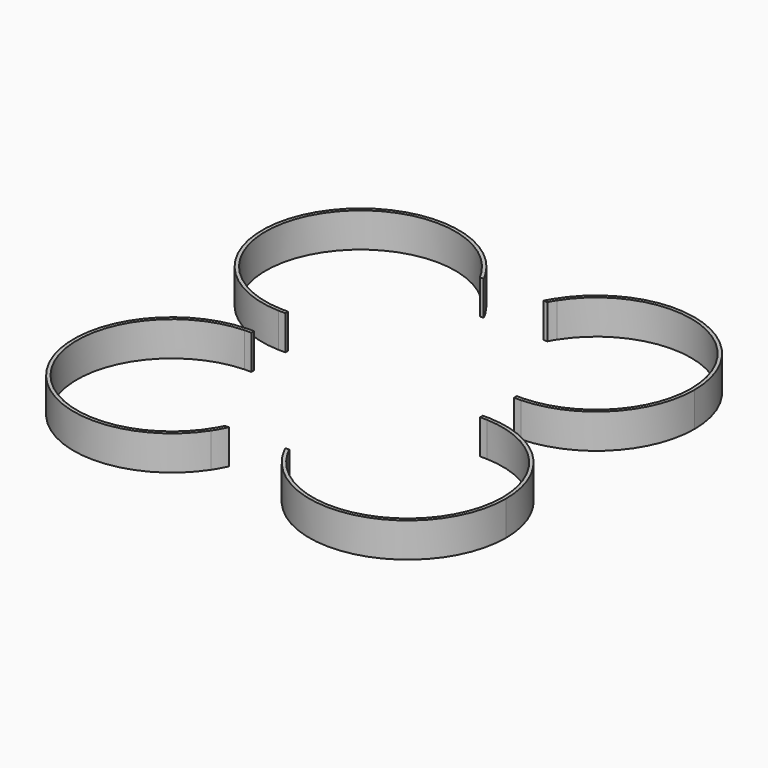
from build123d import *

# Parameters (mm, degrees)
F1_DEPTH = 10


with BuildPart() as f1:
    # F0 (on Top) → F1 (new body)
    with BuildSketch(Plane.XY):
        with BuildLine():
            ThreePointArc((-35.1387531032, -6.6569409359), (-34.1387531032, -6.6387531032), (-33.1387531032, -6.6569409359))
            Line((-33.1387531032, -6.6569409359), (-33.1387531032, -5.6563023659))
            ThreePointArc((-33.1387531032, -5.6563023659), (-34.1387531032, -5.6387531032), (-35.1387531032, -5.6563023659))
            Line((-35.1387531032, -5.6563023659), (-35.1387531032, -6.6569409359))
        make_face()
        with BuildLine():
            Line((-8.2170735426, -45.9842808987), (-9.3207461074, -45.9842808987))
            ThreePointArc((-9.3207461074, -45.9842808987), (-9.8032628947, -46.9463257191), (-10.3230544991, -47.8887531032))
            Line((-10.3230544991, -47.8887531032), (-10.3230544991, -49.7932253077))
            ThreePointArc((-10.3230544991, -49.7932253077), (-9.1972473136, -47.9290137587), (-8.2170735426, -45.9842808987))
        make_face()
        with BuildLine():
            ThreePointArc((-10.3230544991, -47.8887531032), (-57.7004722542, -48.3195637518), (-35.1387531032, -6.6569409359))
            Line((-35.1387531032, -6.6569409359), (-35.1387531032, -5.6563023659))
            ThreePointArc((-35.1387531032, -5.6563023659), (-58.9813781132, -48.1063578589), (-10.3230544991, -49.7932253077))
            Line((-10.3230544991, -49.7932253077), (-10.3230544991, -47.8887531032))
        make_face()
    extrude(amount=F1_DEPTH)


with BuildPart() as f1b:
    # F0 (on Top) → F1, piece 2 (new body)
    with BuildSketch(Plane.XY):
        with BuildLine():
            Line((9.3207461074, -45.9842808987), (8.2170735426, -45.9842808987))
            ThreePointArc((8.2170735426, -45.9842808987), (9.1972473136, -47.9290137587), (10.3230544991, -49.7932253077))
            Line((10.3230544991, -49.7932253077), (10.3230544991, -47.8887531032))
            ThreePointArc((10.3230544991, -47.8887531032), (9.8032628947, -46.9463257191), (9.3207461074, -45.9842808987))
        make_face()
        with BuildLine():
            Line((10.3230544991, -47.8887531032), (10.3230544991, -49.7932253077))
            ThreePointArc((10.3230544991, -49.7932253077), (42.3088996681, -61.4425752735), (62.6387531032, -34.1387531032))
            ThreePointArc((62.6387531032, -34.1387531032), (54.641801657, -14.3429202084), (35.1387531032, -5.6563023659))
            Line((35.1387531032, -5.6563023659), (35.1387531032, -6.6569409359))
            ThreePointArc((35.1387531032, -6.6569409359), (53.934585998, -15.0501439344), (61.6387531032, -34.1387531032))
            ThreePointArc((61.6387531032, -34.1387531032), (41.2562768435, -60.7017133261), (10.3230544991, -47.8887531032))
        make_face()
        with BuildLine():
            Line((35.1387531032, -5.6563023659), (33.1387531032, -5.6563023659))
            Line((33.1387531032, -5.6563023659), (33.1387531032, -6.6569409359))
            ThreePointArc((33.1387531032, -6.6569409359), (34.1387531032, -6.6387531032), (35.1387531032, -6.6569409359))
            Line((35.1387531032, -6.6569409359), (35.1387531032, -5.6563023659))
        make_face()
    extrude(amount=F1_DEPTH)


with BuildPart() as f1c:
    # F0 (on Top) → F1, piece 3 (new body)
    with BuildSketch(Plane.XY):
        with BuildLine():
            Line((-35.1387531032, 5.6563023659), (-33.1387531032, 5.6563023659))
            Line((-33.1387531032, 5.6563023659), (-33.1387531032, 6.6569409359))
            ThreePointArc((-33.1387531032, 6.6569409359), (-34.1387531032, 6.6387531032), (-35.1387531032, 6.6569409359))
            Line((-35.1387531032, 6.6569409359), (-35.1387531032, 5.6563023659))
        make_face()
        with BuildLine():
            ThreePointArc((-9.7525377347, 48.8887531032), (-58.7149604286, 48.5699704287), (-35.1387531032, 5.6563023659))
            Line((-35.1387531032, 5.6563023659), (-35.1387531032, 6.6569409359))
            ThreePointArc((-35.1387531032, 6.6569409359), (-57.996635313, 47.8154287396), (-10.9291107104, 48.8887531032))
            Line((-10.9291107104, 48.8887531032), (-9.7525377347, 48.8887531032))
        make_face()
        with BuildLine():
            ThreePointArc((-8.6497849012, 46.8887531032), (-9.1811193202, 47.8998037881), (-9.7525377347, 48.8887531032))
            Line((-9.7525377347, 48.8887531032), (-10.9291107104, 48.8887531032))
            ThreePointArc((-10.9291107104, 48.8887531032), (-10.3300702173, 47.9008975305), (-9.7730497479, 46.8887531032))
            Line((-9.7730497479, 46.8887531032), (-8.6497849012, 46.8887531032))
        make_face()
    extrude(amount=F1_DEPTH)


with BuildPart() as f1d:
    # F0 (on Top) → F1, piece 4 (new body)
    with BuildSketch(Plane.XY):
        with BuildLine():
            Line((33.1387531032, 6.6569409359), (33.1387531032, 5.6563023659))
            Line((33.1387531032, 5.6563023659), (35.1387531032, 5.6563023659))
            Line((35.1387531032, 5.6563023659), (35.1387531032, 6.6569409359))
            ThreePointArc((35.1387531032, 6.6569409359), (34.1387531032, 6.6387531032), (33.1387531032, 6.6569409359))
        make_face()
        with BuildLine():
            Line((10.9291107104, 48.8887531032), (9.7525377347, 48.8887531032))
            ThreePointArc((9.7525377347, 48.8887531032), (9.1811193202, 47.8998037881), (8.6497849012, 46.8887531032))
            Line((8.6497849012, 46.8887531032), (9.7730497479, 46.8887531032))
            ThreePointArc((9.7730497479, 46.8887531032), (10.3300702173, 47.9008975305), (10.9291107104, 48.8887531032))
        make_face()
        with BuildLine():
            ThreePointArc((62.6387531032, 34.1387531032), (41.7952164512, 61.591049346), (9.7525377347, 48.8887531032))
            Line((9.7525377347, 48.8887531032), (10.9291107104, 48.8887531032))
            ThreePointArc((10.9291107104, 48.8887531032), (41.8194052304, 60.5443885415), (61.6387531032, 34.1387531032))
            ThreePointArc((61.6387531032, 34.1387531032), (53.934585998, 15.0501439344), (35.1387531032, 6.6569409359))
            Line((35.1387531032, 6.6569409359), (35.1387531032, 5.6563023659))
            ThreePointArc((35.1387531032, 5.6563023659), (54.641801657, 14.3429202084), (62.6387531032, 34.1387531032))
        make_face()
    extrude(amount=F1_DEPTH)


solid = Compound([f1.part, f1b.part, f1c.part, f1d.part])
